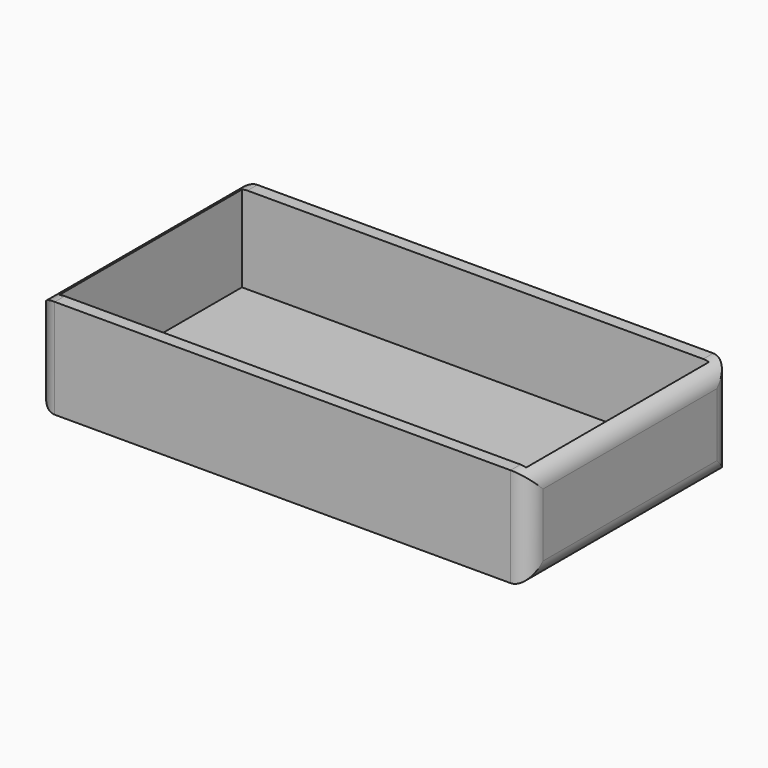
from build123d import *

# Parameters (mm, degrees)
F0_W        = 50.292
F0_H        = 25.908
F1_DEPTH    = 10.16
F2_W        = 47.752
F2_H        = 23.368
F3_DEPTH    = 8.89
F4_T1_DEPTH = 19.3581536726
F4_T3_DEPTH = 35.1061536726
F5_T1_DEPTH = 19.3581536726
F5_T3_DEPTH = 35.1061536726


# Not quite as in the source:
# - a fillet or chamfer that OpenCascade refuses, or shapes differently, is made with other operations: its cross-section is extruded or revolved along the edge and cut away or added
# - a feature names something its author has since deleted; it is built from what else it names


with BuildPart() as f1:
    # F0 (on Top) → F1 (new body)
    with BuildSketch(Plane.XY):
        Rectangle(F0_W, F0_H)
    extrude(amount=F1_DEPTH)

    # F2 (on face) → F3 (cut)
    with BuildSketch(Plane.XY.offset(10.16)):
        Rectangle(F2_W, F2_H)
    extrude(amount=-F3_DEPTH, mode=Mode.SUBTRACT)

    # F4: fillet of radius 1.8396307345 on 4 edges, made by hand

    # F4_s2 → F4_t1 (cut)
    with BuildSketch(Plane.XY.offset(-4.5990768363)):
        with BuildLine():
            ThreePointArc((-23.3063692655, 12.954), (-24.6071846327, 12.4151846327), (-25.146, 11.1143692655))
            Line((-25.146, 11.1143692655), (-25.146, 12.954))
            Line((-25.146, 12.954), (-23.3063692655, 12.954))
        make_face()
        with BuildLine():
            ThreePointArc((-25.146, -11.1143692655), (-24.6071846327, -12.4151846327), (-23.3063692655, -12.954))
            Line((-23.3063692655, -12.954), (-25.146, -12.954))
            Line((-25.146, -12.954), (-25.146, -11.1143692655))
        make_face()
    extrude(amount=F4_T1_DEPTH, mode=Mode.SUBTRACT)

    # F4_s4 → F4_t3 (cut)
    with BuildSketch(Plane.XZ.offset(-17.5530768363)):
        with BuildLine():
            ThreePointArc((-25.146, 1.8396307345), (-24.6071846327, 0.5388153673), (-23.3063692655, 0))
            Line((-23.3063692655, 0), (-25.146, 0))
            Line((-25.146, 0), (-25.146, 1.8396307345))
        make_face()
        with BuildLine():
            ThreePointArc((-25.146, 8.3203692655), (-24.6071846327, 9.6211846327), (-23.3063692655, 10.16))
            Line((-23.3063692655, 10.16), (-25.146, 10.16))
            Line((-25.146, 10.16), (-25.146, 8.3203692655))
        make_face()
    extrude(amount=F4_T3_DEPTH, mode=Mode.SUBTRACT)

    # F5: fillet of radius 1.8396307345 on 4 edges, made by hand

    # F5_s2 → F5_t1 (cut)
    with BuildSketch(Plane.XY.offset(-4.5990768363)):
        with BuildLine():
            ThreePointArc((25.146, -11.1143692655), (24.6071846327, -12.4151846327), (23.3063692655, -12.954))
            Line((23.3063692655, -12.954), (25.146, -12.954))
            Line((25.146, -12.954), (25.146, -11.1143692655))
        make_face()
        with BuildLine():
            ThreePointArc((23.3063692655, 12.954), (24.6071846327, 12.4151846327), (25.146, 11.1143692655))
            Line((25.146, 11.1143692655), (25.146, 12.954))
            Line((25.146, 12.954), (23.3063692655, 12.954))
        make_face()
    extrude(amount=F5_T1_DEPTH, mode=Mode.SUBTRACT)

    # F5_s4 → F5_t3 (cut)
    with BuildSketch(Plane.XZ.offset(-17.5530768363)):
        with BuildLine():
            ThreePointArc((23.3063692655, 0), (24.6071846327, 0.5388153673), (25.146, 1.8396307345))
            Line((25.146, 1.8396307345), (25.146, 0))
            Line((25.146, 0), (23.3063692655, 0))
        make_face()
        with BuildLine():
            ThreePointArc((23.3063692655, 10.16), (24.6071846327, 9.6211846327), (25.146, 8.3203692655))
            Line((25.146, 8.3203692655), (25.146, 10.16))
            Line((25.146, 10.16), (23.3063692655, 10.16))
        make_face()
    extrude(amount=F5_T3_DEPTH, mode=Mode.SUBTRACT)


solid = f1.part
